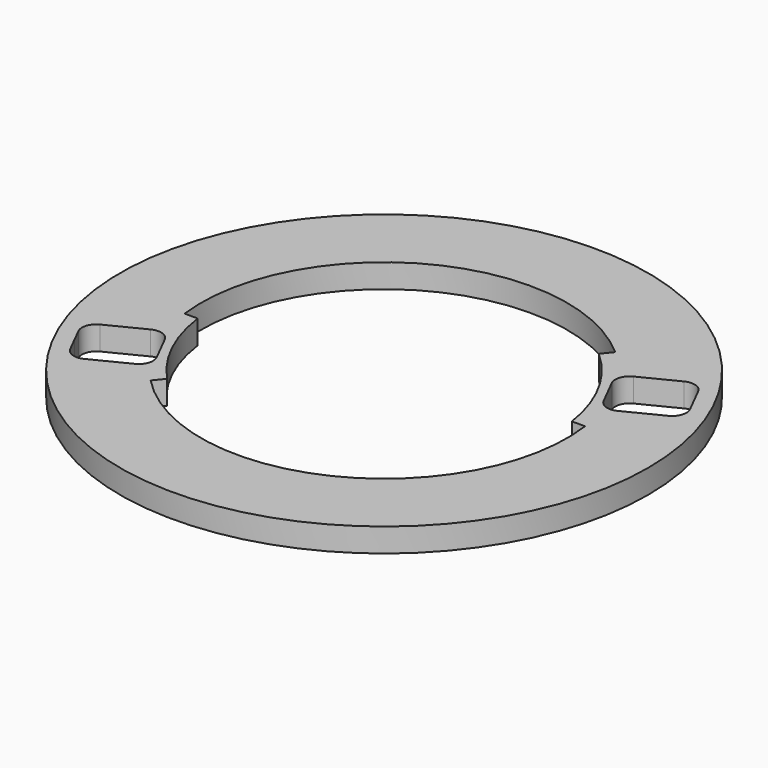
from build123d import *

# Parameters (mm, degrees)
F0_R     = 55.5
F1_DEPTH = 5
F2_R     = 3


with BuildPart() as f1:
    # F0 (on Top) → F1 (new body)
    with BuildSketch(Plane.XY):
        Circle(F0_R)
        Polygon((-43.6709144021, -28.8896496715), (-46.4835835158, -23.3083064231), (-49.2962526295, -17.7269631746), (-36.3475362931, -11.2015708309), (-30.7221980657, -22.3642573278), align=None, mode=Mode.SUBTRACT)
        with BuildLine():
            ThreePointArc((-25.9631257504, -24.5759761), (-32.2743582607, -15.3762251173), (-35.4424777104, -4.6790248716))
            Line((-35.4424777104, -4.6790248716), (-38.2146140403, -4.6790248716))
            ThreePointArc((-38.2146140403, -4.6790248716), (-17.8953589694, 34.0882109733), (25.553195754, 28.797294782))
            Line((25.553195754, 28.797294782), (23.8329245146, 26.6468423848))
            ThreePointArc((23.8329245146, 26.6468423848), (31.5030749277, 16.9002594685), (35.381527976, 5.1195681537))
            Line((35.381527976, 5.1195681537), (38.1580924827, 5.1195681537))
            ThreePointArc((38.1580924827, 5.1195681537), (16.7555959393, -34.6626600929), (-27.7152221959, -26.7229575203))
            Line((-27.7152221959, -26.7229575203), (-25.9631257504, -24.5759761))
        make_face(mode=Mode.SUBTRACT)
        Polygon((43.5800816552, 29.0698943851), (46.3897934183, 23.4944195798), (46.3927507689, 23.4885511366), (47.6104286529, 21.0722419435), (49.2024625319, 17.9130763314), (36.2537461955, 11.3876839877), (30.6313653188, 22.5445020413), align=None, mode=Mode.SUBTRACT)
    extrude(amount=F1_DEPTH)

    # F2
    f2_edges = [f1.edges().sort_by_distance(p)[0] for p in [
        (-36.347536, -11.201571, 2.5),
        (-49.296253, -17.726963, 2.5),
        (-30.722198, -22.364257, 2.5),
        (-43.670914, -28.88965, 2.5),
        (36.253746, 11.387684, 2.5),
        (30.631365, 22.544502, 2.5),
        (43.580082, 29.069894, 2.5),
        (49.202463, 17.913076, 2.5),
    ]]
    fillet(f2_edges, radius=F2_R)


solid = f1.part
